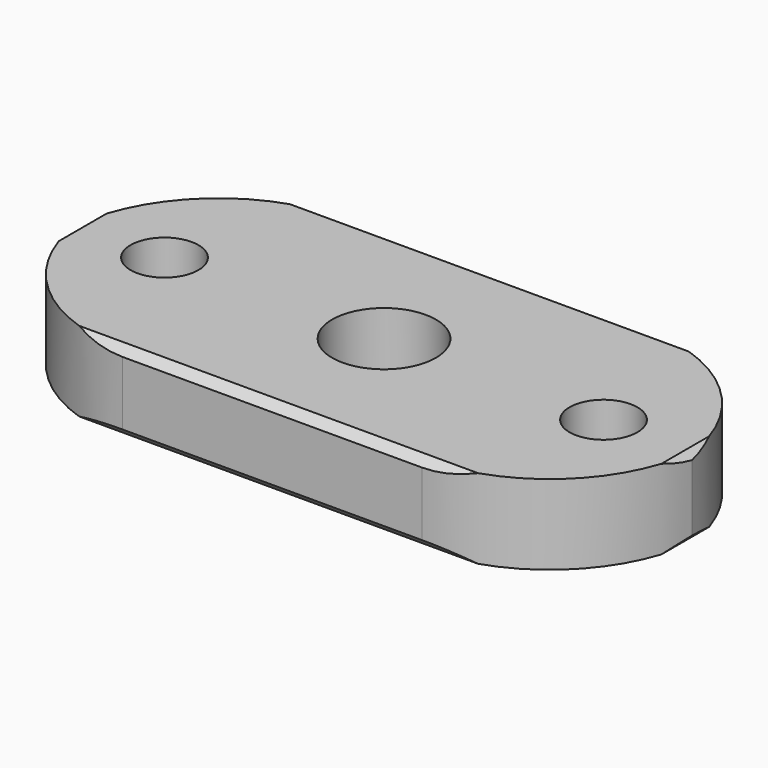
from build123d import *

# Parameters (mm, degrees)
F0_W        = 31
F0_H        = 14
F0_R        = 1.7
F1_DEPTH    = 4
F2_SIZE     = 0.4
F3_T1_DEPTH = 43.2


# Not quite as in the source:
# - a fillet or chamfer that OpenCascade refuses, or shapes differently, is made with other operations: its cross-section is extruded or revolved along the edge and cut away or added


with BuildPart() as f1:
    # F0 (on Top) → F1 (new body)
    with BuildSketch(Plane.XY):
        Rectangle(F0_W, F0_H)
        with Locations((-11, 0)):
            Circle(F0_R, mode=Mode.SUBTRACT)
        with BuildLine():
            ThreePointArc((-2.6, 0), (0, 2.6), (2.6, 0))
            ThreePointArc((2.6, 0), (0, -2.6), (-2.6, 0))
        make_face(mode=Mode.SUBTRACT)
        with Locations((11, 0)):
            Circle(F0_R, mode=Mode.SUBTRACT)
    extrude(amount=F1_DEPTH)

    # F2
    f2_edges = [f1.edges().sort_by_distance(p)[0] for p in [
        (0, -7, 0),
        (0, -7, 4),
        (15.5, 0, 0),
        (15.5, 0, 4),
        (0, 7, 0),
        (0, 7, 4),
        (-15.5, 0, 4),
        (-15.5, 0, 0),
    ]]
    chamfer(f2_edges, length=F2_SIZE)

    # F3: fillet of radius 8 on 4 edges, made by hand

    # F3_s2 → F3_t1 (cut)
    with BuildSketch(Plane.XY.offset(-19.6)):
        with BuildLine():
            ThreePointArc((-7.5, 7), (-13.1568542495, 4.6568542495), (-15.5, -1))
            Line((-15.5, -1), (-15.5, 7))
            Line((-15.5, 7), (-7.5, 7))
        make_face()
        with BuildLine():
            ThreePointArc((-7.5, -7), (-13.1568542495, -4.6568542495), (-15.5, 1))
            Line((-15.5, 1), (-15.5, -7))
            Line((-15.5, -7), (-7.5, -7))
        make_face()
        with BuildLine():
            ThreePointArc((15.5, -1), (13.1568542495, 4.6568542495), (7.5, 7))
            Line((7.5, 7), (15.5, 7))
            Line((15.5, 7), (15.5, -1))
        make_face()
        with BuildLine():
            ThreePointArc((15.5, 1), (13.1568542495, -4.6568542495), (7.5, -7))
            Line((7.5, -7), (15.5, -7))
            Line((15.5, -7), (15.5, 1))
        make_face()
    extrude(amount=F3_T1_DEPTH, mode=Mode.SUBTRACT)


solid = f1.part
